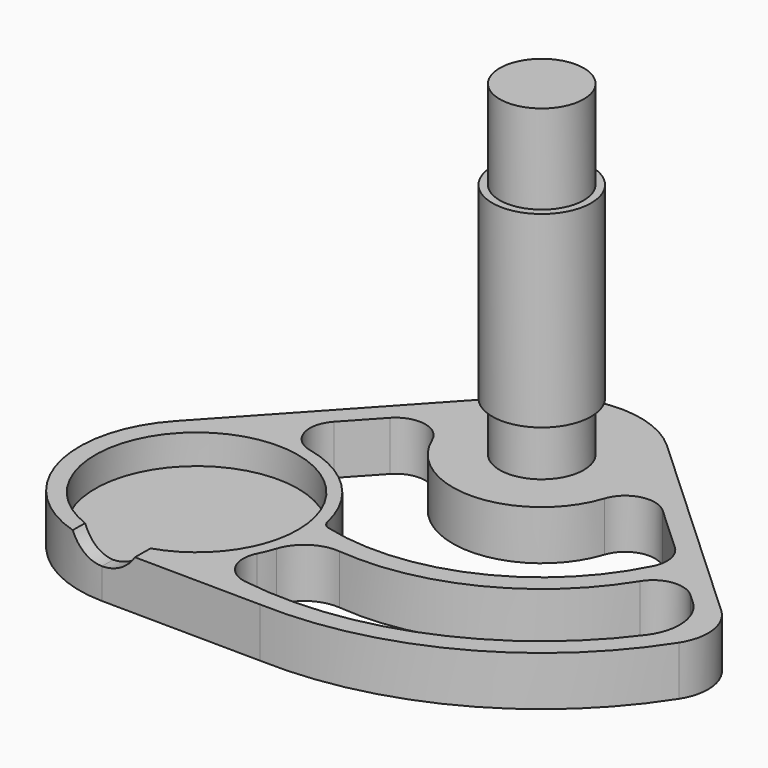
from build123d import *

# Parameters (mm, degrees)
F0_R     = 10.25
F0_R_2   = 5
F0_R_3   = 4.25
F1_DEPTH = 5
F2_DEPTH = 33
F3_DEPTH = 24
F4_DEPTH = 3
F5_DEPTH = 5
F7_DEPTH = 2.0316230768


# Not quite as in the source:
# - a feature names something its author has since deleted; it is built from what else it names


with BuildPart() as f1:
    # F0 (on Top) → F1 (new body)
    with BuildSketch(Plane.XY):
        with BuildLine():
            ThreePointArc((37.8886156331, -47.7045562268), (30.7058016888, -45.0614846038), (23.757851373, -48.271567184))
            Line((23.757851373, -48.271567184), (4.9458403192, -68.6563901516))
            ThreePointArc((4.9458403192, -68.6563901516), (2.7469798041, -81.5500736227), (13.6377095304, -88.793972231))
            Line((13.6377095304, -88.793972231), (29.73595993, -88.9640810988))
            ThreePointArc((29.73595993, -88.9640810988), (46.7599967293, -85.1663293947), (59.6493608288, -73.4145193188))
            ThreePointArc((59.6493608288, -73.4145193188), (60.4040648618, -70.0765035789), (58.8352277111, -67.0350109763))
            Line((58.8352277111, -67.0350109763), (37.8886156331, -47.7045562268))
        make_face()
        with Locations((13.8766520367, -77.1243319886)):
            Circle(F0_R, mode=Mode.SUBTRACT)
        with BuildLine():
            ThreePointArc((26.3755166306, -86.6270533164), (24.155278042, -85.0381292254), (24.1421413752, -82.307933887))
            ThreePointArc((24.1421413752, -82.307933887), (24.5057243444, -81.5144142062), (24.808075333, -80.6956041311))
            ThreePointArc((24.808075333, -80.6956041311), (26.4141385233, -78.5946086732), (28.9801509243, -77.9549202777))
            ThreePointArc((28.9801509243, -77.9549202777), (41.3836815678, -75.6297518396), (50.6933671902, -67.110143028))
            ThreePointArc((50.6933671902, -67.110143028), (52.8388421265, -65.7108085683), (55.2827077781, -66.4780896835))
            Line((55.2827077781, -66.4780896835), (56.196743854, -67.321602369))
            ThreePointArc((56.196743854, -67.321602369), (57.7828175357, -70.5171396289), (56.835176405, -73.9564803202))
            ThreePointArc((56.835176405, -73.9564803202), (43.3687378078, -84.5309041293), (26.3755166306, -86.6270533164))
        make_face(mode=Mode.SUBTRACT)
        with BuildLine():
            ThreePointArc((17.829474896, -57.6446324429), (20.5558252215, -56.7249026703), (22.8022906293, -58.5227575376))
            ThreePointArc((22.8022906293, -58.5227575376), (31.4675825452, -64.046207144), (39.6624601723, -57.8462264813))
            ThreePointArc((39.6624601723, -57.8462264813), (41.7576536692, -55.8741582362), (44.5489302313, -56.5724877473))
            Line((44.5489302313, -56.5724877473), (49.2396549007, -60.901294746))
            ThreePointArc((49.2396549007, -60.901294746), (50.1561683514, -62.5663798864), (49.8881507259, -64.4480472275))
            ThreePointArc((49.8881507259, -64.4480472275), (39.7927356809, -74.1728962685), (25.8272247035, -75.3789629921))
            ThreePointArc((25.8272247035, -75.3789629921), (25.3591431783, -75.10558707), (25.1024718967, -74.6281411964))
            ThreePointArc((25.1024718967, -74.6281411964), (22.0019832723, -68.9862122849), (16.3551853155, -65.8946003451))
            ThreePointArc((16.3551853155, -65.8946003451), (14.1394417768, -63.8635142203), (14.7970929317, -60.9305421383))
            Line((14.7970929317, -60.9305421383), (17.829474896, -57.6446324429))
        make_face(mode=Mode.SUBTRACT)
        with Locations((31.1067389816, -55.0534438355)):
            Circle(F0_R_2, mode=Mode.SUBTRACT)
        with Locations((13.8766520367, -77.1243319886)):
            Circle(F0_R)
        with Locations((31.1067389816, -55.0534438355)):
            Circle(F0_R_2)
        with Locations((31.1067389816, -55.0534438355)):
            Circle(F0_R_3, mode=Mode.SUBTRACT)
    extrude(amount=-F1_DEPTH)



with BuildPart() as f2:
    # F0 (on Top) → F2 (new body)
    with BuildSketch(Plane.XY):
        with Locations((31.1067389816, -55.0534438355)):
            Circle(F0_R_3)
    extrude(amount=F2_DEPTH)


with BuildPart() as f1_1:
    add(f1.part)

    add(f2.part)  # F3 merges F2
    # F0 (on Top) → F3 (join)
    with BuildSketch(Plane.XY):
        with Locations((31.1067389816, -55.0534438355)):
            Circle(F0_R_2)
        with Locations((31.1067389816, -55.0534438355)):
            Circle(F0_R_3, mode=Mode.SUBTRACT)
    extrude(amount=F3_DEPTH)

    # F0 (on Top) → F4 (cut)
    with BuildSketch(Plane.XY):
        with Locations((13.8766520367, -77.1243319886)):
            Circle(F0_R)
    extrude(amount=-F4_DEPTH, mode=Mode.SUBTRACT)

    # F0 (on Top) → F5 (cut)
    with BuildSketch(Plane.XY):
        with Locations((31.1067389816, -55.0534438355)):
            Circle(F0_R_2)
        with Locations((31.1067389816, -55.0534438355)):
            Circle(F0_R_3, mode=Mode.SUBTRACT)
    extrude(amount=F5_DEPTH, mode=Mode.SUBTRACT)

    # F6 (on face) → F7 (cut, through all)
    with BuildSketch(Plane(origin=(-0.9366511213, -88.639966179, 0), x_dir=(0.9999441748, -0.0105663266, 0), z_dir=(-0.0105663266, -0.9999441748, 0))):
        with BuildLine():
            Line((14.5751743135, -1.9074911252), (14.5751743135, 0))
            Line((14.5751743135, 0), (11.210032617, 0))
            ThreePointArc((11.210032617, 0), (12.6485346529, -1.384324833), (14.5751743135, -1.9074911252))
        make_face()
        with BuildLine():
            ThreePointArc((14.5751743135, -1.9074911252), (16.501813974, -1.384324833), (17.94031601, 0))
            Line((17.94031601, 0), (14.5751743135, 0))
            Line((14.5751743135, 0), (14.5751743135, -1.9074911252))
        make_face()
    extrude(amount=-F7_DEPTH, mode=Mode.SUBTRACT)


solid = f1_1.part
